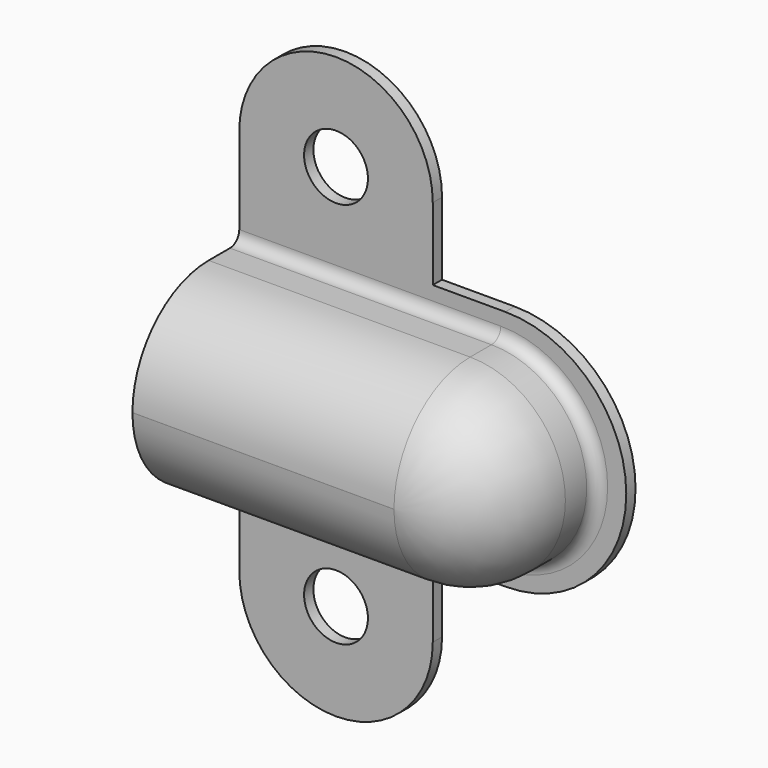
from build123d import *

# Parameters (mm, degrees)
F1_DEPTH    = 0.762
F3_DEPTH    = 8.763
F4_R        = 6.2484
F5_R        = 2.0955
F6_DEPTH    = 0.763
F7_T        = 0.762
F7_T3_DEPTH = 18.68884375
F7_T5_DEPTH = 2.286
F7_T8_ANGLE = 180.000000001
F8_DEPTH    = 0.763
F9_R        = 0.762


# Not quite as in the source:
# - a shell that OpenCascade refuses in one call is made with other operations: the cavity is built on its own and cut out


with BuildPart() as f1:
    # F0 (on Front) → F1 (new body)
    with BuildSketch(Plane.XZ):
        with BuildLine():
            ThreePointArc((12.7, 12.7), (6.35, 19.05), (0, 12.7))
            Line((0, 12.7), (0, -12.7))
            ThreePointArc((0, -12.7), (6.35, -19.05), (12.7, -12.7))
            Line((12.7, -12.7), (12.7, -7.9375))
            Line((12.7, -7.9375), (17.4625, -7.9375))
            ThreePointArc((17.4625, -7.9375), (25.4, 0), (17.4625, 7.9375))
            Line((17.4625, 7.9375), (12.7, 7.9375))
            Line((12.7, 7.9375), (12.7, 12.7))
        make_face()
    extrude(amount=-F1_DEPTH)

    # F2 (on face) → F3 (join)
    with BuildSketch(Plane.XZ):
        with BuildLine():
            Line((17.16484375, 6.25078125), (0, 6.25078125))
            Line((0, 6.25078125), (0, -6.25078125))
            Line((0, -6.25078125), (17.16484375, -6.25078125))
            ThreePointArc((17.16484375, -6.25078125), (23.415625, 0), (17.16484375, 6.25078125))
        make_face()
    extrude(amount=F3_DEPTH)

    # F4
    f4_edges = [f1.edges().sort_by_distance(p)[0] for p in [
        (8.582422, -8.763, 6.250781),
    ]]
    fillet(f4_edges, radius=F4_R)

    # F5 (on face) → F6 (cut, through all)
    with BuildSketch(Plane.XZ):
        with Locations((6.35, 12.7)):
            Circle(F5_R)
        with Locations((6.35, -12.7)):
            Circle(F5_R)
    extrude(amount=-F6_DEPTH, mode=Mode.SUBTRACT)

    # F7: shell of thickness 0.762, made by hand


with BuildPart() as f7_core1:
    # F7_t2: copy of F1
    add(f1.part)

    # the walls: a layer under each face that stays
    f7_faces = [f7_core1.faces().sort_by_distance(p)[0] for p in [
        (8.582421875, -1.2573, -6.25078125),
        (8.582421875, -6.9328860116, -4.4206672616),
        (4.2333333333, 0, -12.7),
        (8.5836125, -8.763, 0),
        (6.35, 0.381, -19.05),
        (8.582421875, -6.9328860116, 4.4206672616),
        (12.7, 0.762, 0),
        (8.582421875, -1.2573, 6.25078125),
        (6.35, 0.381, 19.05),
        (23.415625, -1.2573, 0),
        (21.5855110116, -6.9328860116, 0),
        (12.7, 0.381, -10.31875),
        (15.08125, 0.381, -7.9375),
        (25.4, 0.381, 0),
        (15.08125, 0.381, 7.9375),
        (12.7, 0.381, 10.31875),
        (4.2545, 0.381, -12.7),
        (4.2545, 0.381, 12.7),
    ]]
    thicken(f7_faces, amount=-F7_T, mode=Mode.SUBTRACT)

    # F7_s4 → F7_t3 (cut)
    with BuildSketch(Plane.YZ.offset(-0.762)):
        Polygon((-0.00762, -6.25840125), (0, -5.48878125), (0.762, -5.48878125), (0.762, -6.25078125), align=None)
        Polygon((-0.00762, 6.25840125), (0.762, 6.25078125), (0.762, 5.48878125), (0, 5.48878125), align=None)
    extrude(amount=F7_T3_DEPTH, mode=Mode.SUBTRACT)

    # F7_s6 → F7_t5 (cut)
    with BuildSketch(Plane.XZ.offset(-1.524)):
        Polygon((12.70762, -7.94512), (11.938, -7.9375), (11.938, -7.1755), (12.7, -7.1755), align=None)
        Polygon((12.70762, 7.94512), (12.7, 7.1755), (11.938, 7.1755), (11.938, 7.9375), align=None)
    extrude(amount=F7_T5_DEPTH, mode=Mode.SUBTRACT)

    # F7_s7 → F7_t8 (revolve, cut)
    with BuildSketch(Plane.YZ.offset(17.16484375)):
        Polygon((-0.00762, -6.25840125), (0.762, -6.25078125), (0.762, -5.48878125), (0, -5.48878125), align=None)
    revolve(axis=Axis((17.16484375, 0, 0), (0, -1, 0)), revolution_arc=F7_T8_ANGLE, mode=Mode.SUBTRACT)


with BuildPart() as f1_1:
    add(f1.part)

    # what is left inside the walls is the cavity
    f7_cavity = [f7_core1.part.solids().sort_by_distance(p)[0] for p in [
        (11.326812, -0.00762, -1.829594),
    ]]
    add(f7_cavity, mode=Mode.SUBTRACT)

    # F8 (cut, through all): a face of the model
    f8_faces = [f1_1.faces().sort_by_distance(p)[0] for p in [
        (10.7728031168, 0, 0),
    ]]
    extrude(f8_faces, amount=-F8_DEPTH, mode=Mode.SUBTRACT)

    # F9
    f9_edges = [f1_1.edges().sort_by_distance(p)[0] for p in [
        (8.582422, 0, 6.250781),
        (8.582422, 0.762, 5.488781),
    ]]
    fillet(f9_edges, radius=F9_R)


solid = f1_1.part
